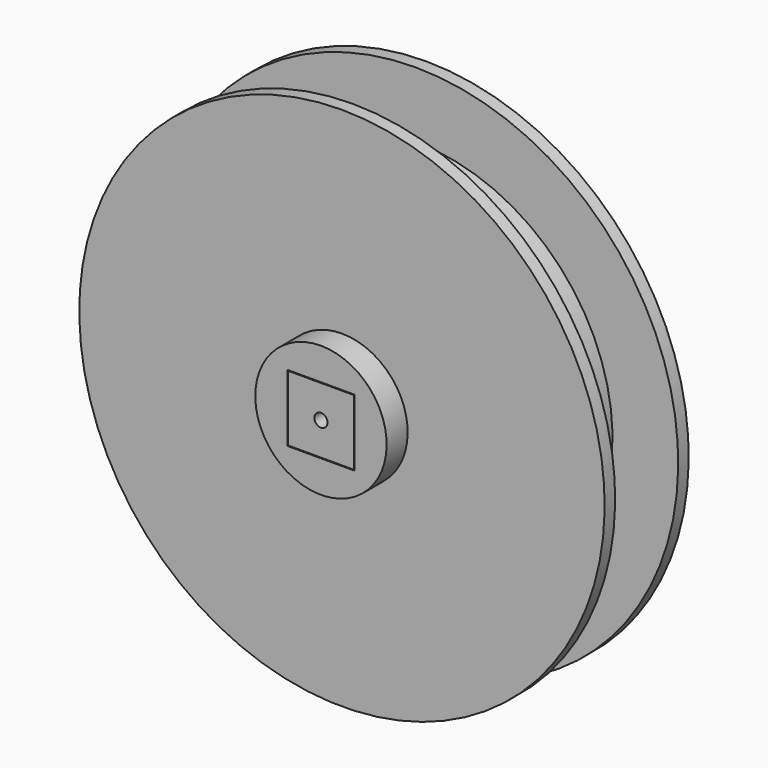
from build123d import *

# Parameters (mm, degrees)
F0_W     = 15
F0_H     = 15
F0_R     = 1.5
F1_DEPTH = 30
F3_D     = 3.3
F3_DEPTH = 8
F3_TIP   = 0.9914200214
F6_W     = 15.3
F6_H     = 15.3
F7_DEPTH = 30.0010001


with BuildPart() as f1:
    # F0 (on Front) → F1 (new body)
    with BuildSketch(Plane.XZ):
        Rectangle(F0_W, F0_H)
        Circle(F0_R, mode=Mode.SUBTRACT)
    extrude(amount=F1_DEPTH)

    # F3
    with Locations(Plane.XY.offset(7.5)):
        with Locations((0, -7.4150050059), (0, -23.6950945109)):
            Hole(F3_D / 2, depth=F3_DEPTH)
            with Locations((0, 0, -(F3_DEPTH + F3_TIP / 2))):  # 118° drill point
                Cone(0, F3_D / 2, F3_TIP, mode=Mode.SUBTRACT)


with BuildPart() as f5:
    # F4 (on Right) → F5 (revolve)
    with BuildSketch(Plane.YZ):
        Polygon((-30, 0), (0, 0), (0, 60), (-3, 60), (-3, 45), (-21, 45), (-21, 60), (-24, 60), (-24, 15), (-30, 15), align=None)
    revolve(axis=Axis((0, -24.8045190237, 0), (0, 1, 0)))

    # F6 (on Front) → F7 (cut, through all)
    with BuildSketch(Plane.XZ):
        Rectangle(F6_W, F6_H)
    extrude(amount=F7_DEPTH, mode=Mode.SUBTRACT)


solid = Compound([f1.part, f5.part])
